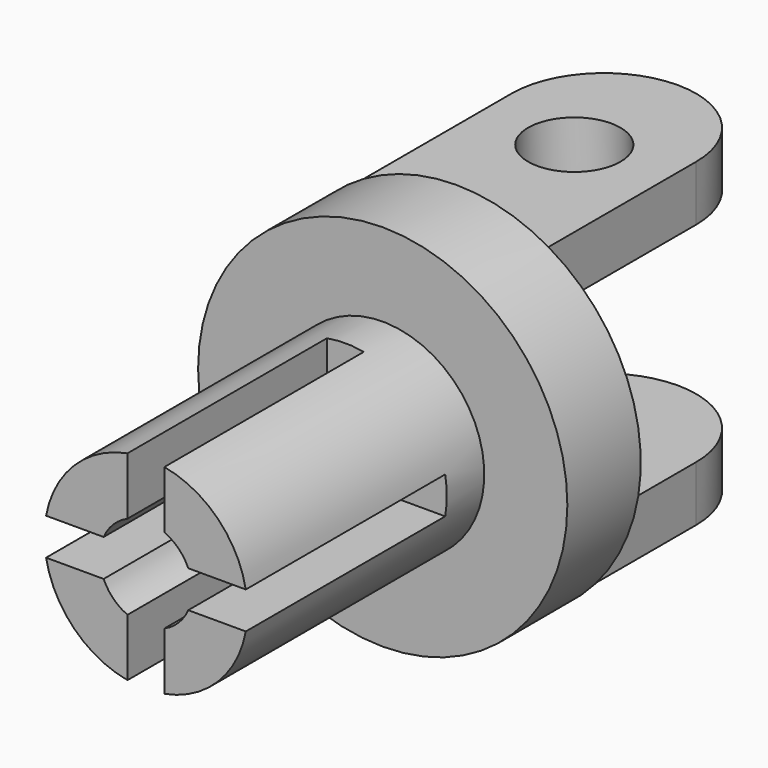
from build123d import *

# Parameters (mm, degrees)
F2_W     = 10
F2_H     = 3
F3_DEPTH = 15
F4_R     = 4.99999
F5_R     = 2.5
F6_DEPTH = 18.6612540378
F7_W     = 2
F7_H     = 5
F7_W_2   = 5
F7_H_2   = 2
F8_DEPTH = 13.5


# Not quite as in the source:
# - a fillet or chamfer is up to 0.001 mm smaller than in the source, because OpenCascade refuses the exact size


with BuildPart() as f1:
    # F0 (on Top) → F1 (revolve)
    with BuildSketch(Plane.XY):
        Polygon((0, 6.2748147342), (-10, 6.2748147342), (-10, 1.304778154), (-5.5, 1.304778154), (-5.5, -14.7251852658), (-2.5, -14.7251852658), (-2.5, 1.2748147342), (0, 1.2748147342), align=None)
    revolve(axis=Axis((0, 3.7748147342, 0), (0, -1, 0)))

    # F2 (on face) → F3 (join)
    with BuildSketch(Plane(origin=(0, 6.2748147342, 0), x_dir=(-1, 0, 0), z_dir=(0, 1, 0))):
        with Locations((0, 7.1602540378)):
            Rectangle(F2_W, F2_H)
        with Locations((0, -7.1602540378)):
            Rectangle(F2_W, F2_H)
    extrude(amount=F3_DEPTH)

    # F4 (radius 5 in the source; OpenCascade refuses exactly that, so slightly less here)
    f4_edges = [f1.edges().sort_by_distance(p)[0] for p in [
        (-5, 21.274815, -7.160254),
        (5, 21.274815, -7.160254),
        (5, 21.274815, 7.160254),
        (-5, 21.274815, 7.160254),
    ]]
    fillet(f4_edges, radius=F4_R)

    # F5 (on face) → F6 (cut, through all)
    with BuildSketch(Plane(origin=(0, 0, -8.6602540378), x_dir=(1, 0, 0), z_dir=(0, 0, -1))):
        with Locations((0, -14.2748147342)):
            Circle(F5_R)
    extrude(amount=-F6_DEPTH, mode=Mode.SUBTRACT)

    # F7 (on face) → F8 (cut)
    with BuildSketch(Plane.XZ.offset(14.7251852658)):
        with Locations((0, 3.7191687186)):
            Rectangle(F7_W, F7_H)
        with Locations((-3.7191687186, 0)):
            Rectangle(F7_W_2, F7_H_2)
        with Locations((0, -3.7191687186)):
            Rectangle(F7_W, F7_H)
        with Locations((3.7191687186, 0)):
            Rectangle(F7_W_2, F7_H_2)
    extrude(amount=-F8_DEPTH, mode=Mode.SUBTRACT)


solid = f1.part
